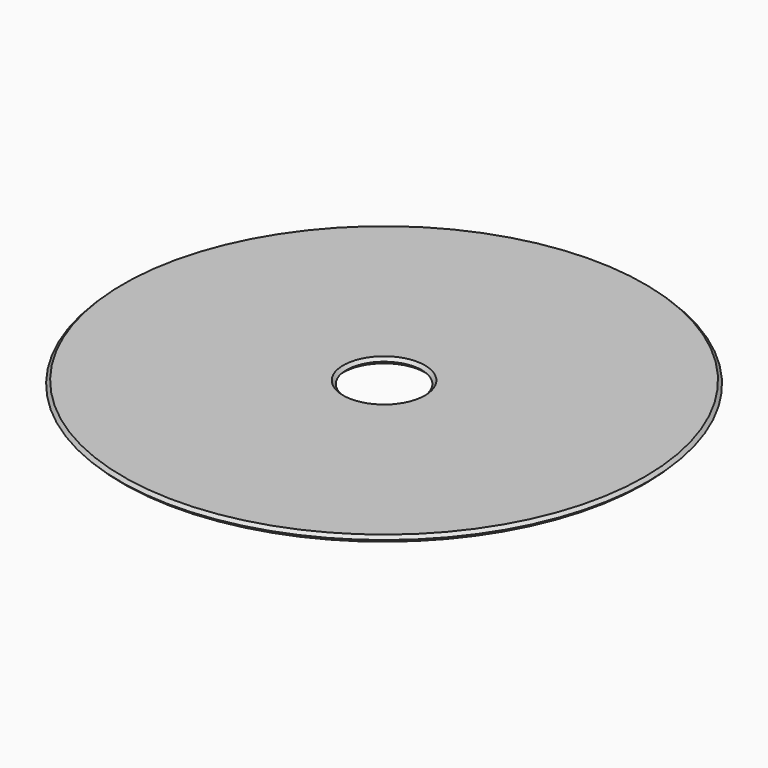
from build123d import *

# Parameters (mm, degrees)
F0_R     = 42
F0_R_2   = 6
F1_DEPTH = 1
F2_SIZE  = 0.49999


# Not quite as in the source:
# - a fillet or chamfer is up to 0.001 mm smaller than in the source, because OpenCascade refuses the exact size


with BuildPart() as f1:
    # F0 (on Top) → F1 (new body)
    with BuildSketch(Plane.XY):
        Circle(F0_R)
        Circle(F0_R_2, mode=Mode.SUBTRACT)
    extrude(amount=F1_DEPTH)

    # F2 (size 0.5 in the source; OpenCascade refuses exactly that, so slightly less here)
    f2_edges = [f1.edges().sort_by_distance(p)[0] for p in [
        (-6, 0, 1),
        (-42, 0, 1),
        (-42, 0, 0),
        (-6, 0, 0),
    ]]
    chamfer(f2_edges, length=F2_SIZE)


solid = f1.part
